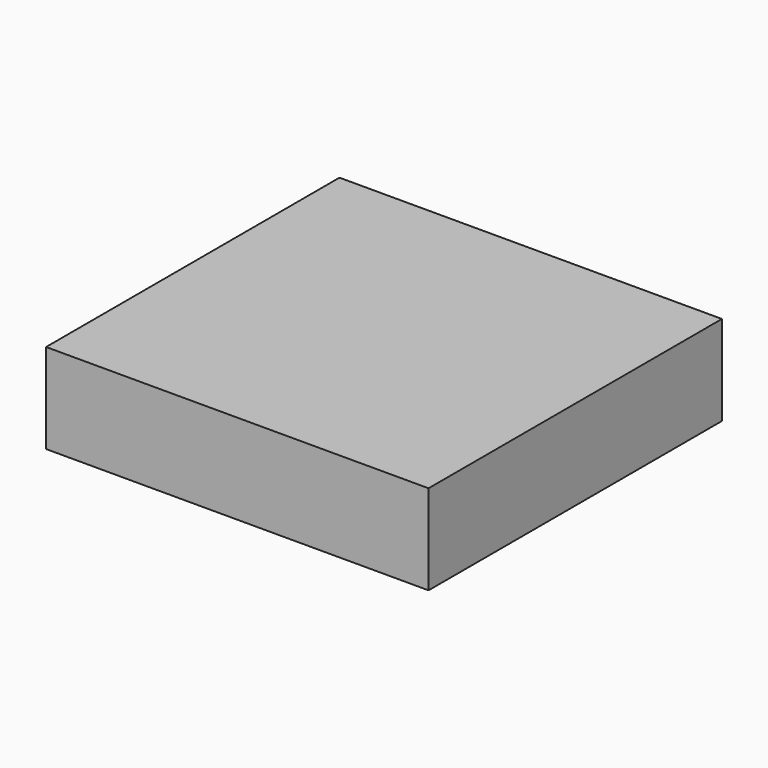
from build123d import *

# Parameters (mm, degrees)
F0_W     = 108.1059202552
F0_H     = 103.6550737917
F3_DEPTH = 25.4


# Not quite as in the source:
# - the program builds the solid bodies; features that only make, move or delete a surface that nothing else refers to are left out


with BuildPart() as f3:
    # F0 (on Top) → F3 (new body)
    with BuildSketch(Plane.XY):
        with Locations((-0.8189864457, -0.2600532025)):
            Rectangle(F0_W, F0_H)
    extrude(amount=F3_DEPTH)


solid = f3.part
